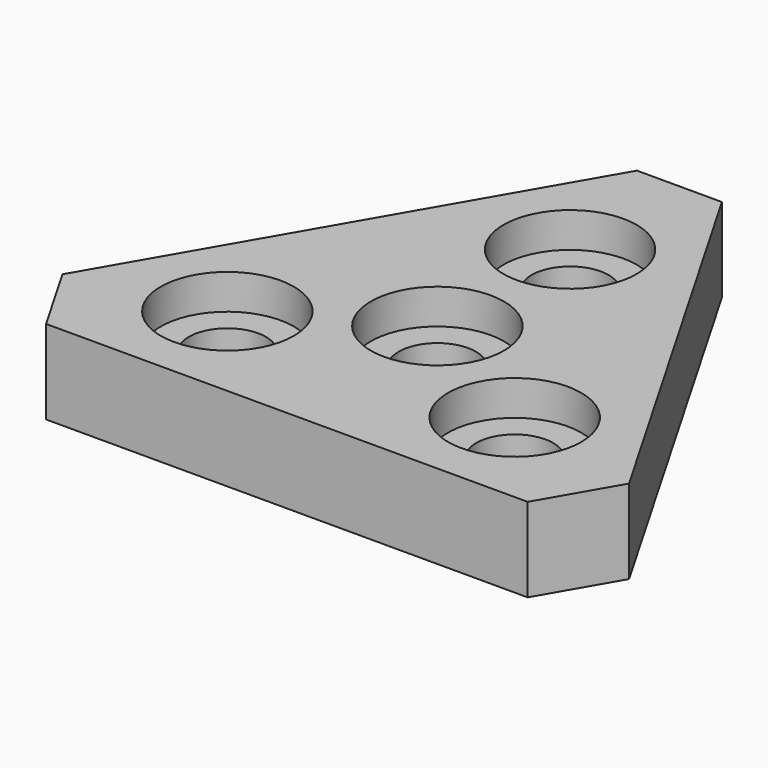
from build123d import *

# Parameters (mm, degrees)
F1_R     = 9.5
F1_R_2   = 5.5
F2_DEPTH = 7
F3_DEPTH = 12


# Not quite as in the source:
# - a feature of the source that left no trace in its solid (it failed there, or was rolled back) is left out


with BuildPart() as f2:
    # F1 (on Top) → F2 (new body)
    with BuildSketch(Plane.XY):
        Polygon((-6.0621778265, 43.1666666667), (-40.4145188433, -16.3333333333), (-34.3523410168, -26.8333333333), (34.3523410168, -26.8333333333), (40.4145188433, -16.3333333333), (6.0621778265, 43.1666666667), align=None)
        with Locations((-20.4959345562, -11.8333333333)):
            Circle(F1_R, mode=Mode.SUBTRACT)
        with Locations((20.4959345562, -11.8333333333)):
            Circle(F1_R, mode=Mode.SUBTRACT)
        Circle(F1_R, mode=Mode.SUBTRACT)
        with Locations((0, 23.6666666667)):
            Circle(F1_R, mode=Mode.SUBTRACT)
        with Locations((0, 23.6666666667)):
            Circle(F1_R)
        with Locations((0, 23.6666666667)):
            Circle(F1_R_2, mode=Mode.SUBTRACT)
        with Locations((-20.4959345562, -11.8333333333)):
            Circle(F1_R)
        with Locations((-20.4959345562, -11.8333333333)):
            Circle(F1_R_2, mode=Mode.SUBTRACT)
        Circle(F1_R)
        Circle(F1_R_2, mode=Mode.SUBTRACT)
        with Locations((20.4959345562, -11.8333333333)):
            Circle(F1_R)
        with Locations((20.4959345562, -11.8333333333)):
            Circle(F1_R_2, mode=Mode.SUBTRACT)
    extrude(amount=F2_DEPTH)

    # F1 (on Top) → F3 (join)
    with BuildSketch(Plane.XY):
        Polygon((-6.0621778265, 43.1666666667), (-40.4145188433, -16.3333333333), (-34.3523410168, -26.8333333333), (34.3523410168, -26.8333333333), (40.4145188433, -16.3333333333), (6.0621778265, 43.1666666667), align=None)
        with Locations((-20.4959345562, -11.8333333333)):
            Circle(F1_R, mode=Mode.SUBTRACT)
        with Locations((20.4959345562, -11.8333333333)):
            Circle(F1_R, mode=Mode.SUBTRACT)
        Circle(F1_R, mode=Mode.SUBTRACT)
        with Locations((0, 23.6666666667)):
            Circle(F1_R, mode=Mode.SUBTRACT)
    extrude(amount=F3_DEPTH)


solid = f2.part
